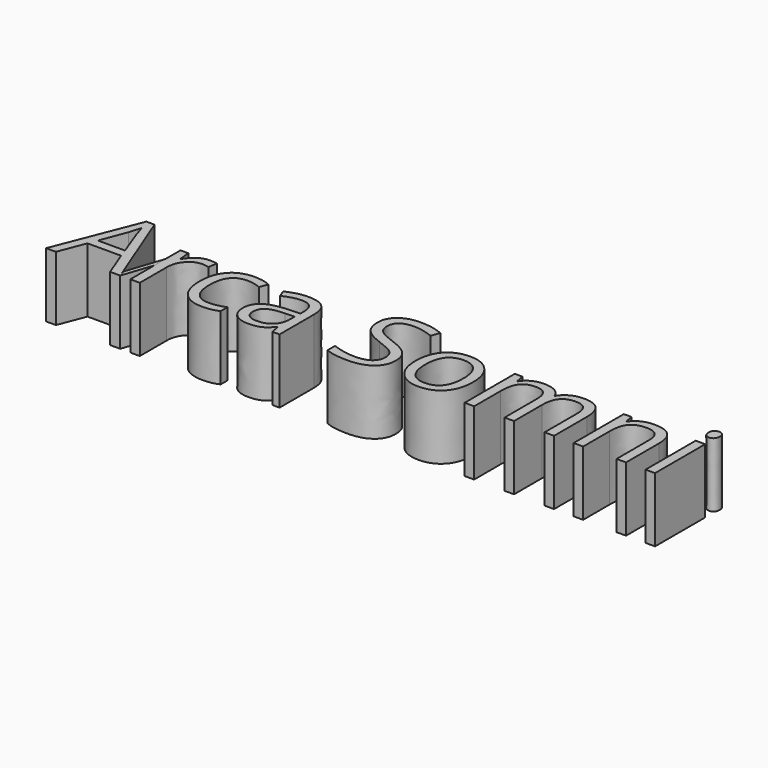
from build123d import *

# Parameters (mm, degrees)
F0_TEXT_SIZE = 46.1281115551
F1_DEPTH     = 25.4
F3_DEPTH     = 25.4


# Not quite as in the source:
# - Text() gives the source's letters only with a copy of the font that has no kerning and outlines rounded to 1/6400 em; it was checked with that copy


with BuildPart() as f1:
    # F0 (on Top) → F1 (new body)
    with BuildSketch(Plane.XY):
        with Locations((-50.6895259023, -4.885149654)):
            Text('Arca Somni', F0_TEXT_SIZE, font='Open Sans', text_align=(TextAlign.LEFT, TextAlign.BOTTOM))
    extrude(amount=-F1_DEPTH)


with BuildPart() as f3:
    # F2 (on Top) → F3 (new body)
    with BuildSketch(Plane.XY):
        Polygon((-22.4078961131, -2.2420807435), (-21.4990803088, -4.885149654), (-17.534945722, 7.0208385587), (-17.534945722, 12.393469248), (-19.3237792701, 7.0208385587), align=None)
    extrude(amount=-F3_DEPTH)


solid = Compound([f1.part, f3.part])
